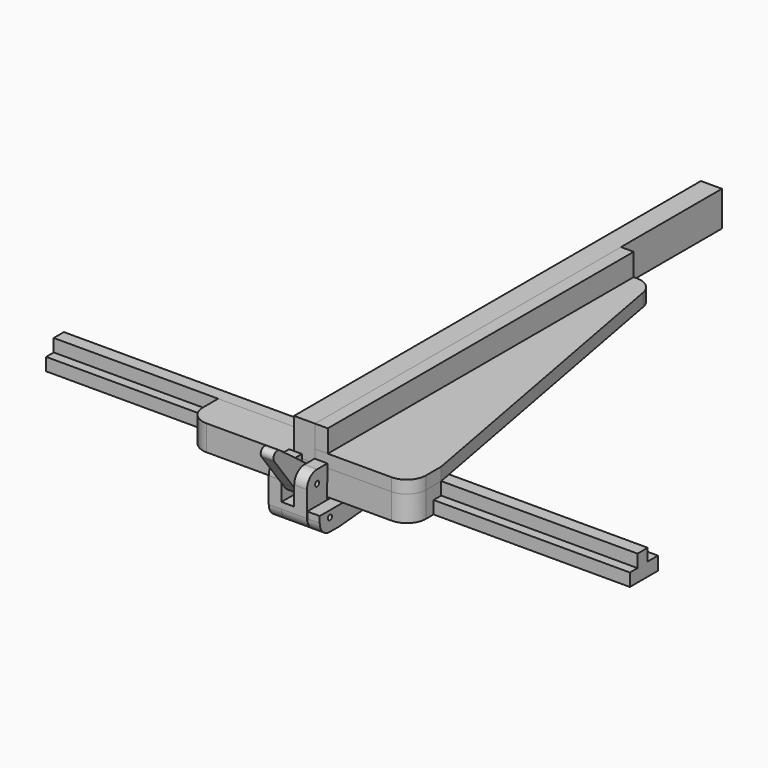
from build123d import *

# Parameters (mm, degrees)
F1_DEPTH      = 798
F2_W          = 150
F2_H          = 15
F3_DEPTH      = 20
F0_W          = 20
F0_H          = 35
F4_DEPTH      = 600
F2_W_2        = 200
F5_DEPTH      = 20
F6_DEPTH      = 40
F8_DEPTH      = 458
F8_DEPTH_BACK = 458
F7_R          = 5.125
F7_R_2        = 4
F9_DEPTH      = 20
F10_DEPTH     = 20
F11_START     = -40
F9_FACE_R     = 5.125
F9_FACE_R_2   = 4
F11_DEPTH     = 20
F12_DEPTH     = 20
F13_START     = 20.5
F13_DEPTH     = 19.5


with BuildPart() as f1:
    # F0 (on Front) → F1 (new body)
    with BuildSketch(Plane.XZ):
        Polygon((-33, 0), (0, 0), (0, 20), (0, 55), (-33, 55), align=None)
    extrude(amount=-F1_DEPTH)


with BuildPart() as f3:
    # F2 (on Top) → F3 (new body)
    with BuildSketch(Plane.XY):
        with BuildLine():
            Line((0, 600), (0, 60))
            Line((0, 60), (150, 60))
            Line((150, 60), (54.5439485545, 575.4626778055))
            ThreePointArc((54.5439485545, 575.4626778055), (44.2303739381, 593.0638281099), (25.045488405, 600))
            Line((25.045488405, 600), (0, 600))
        make_face()
        with BuildLine():
            Line((0, 45), (0, 0))
            Line((0, 0), (120, 0))
            ThreePointArc((120, 0), (141.2132034356, 8.7867965644), (150, 30))
            Line((150, 30), (150, 45))
            Line((150, 45), (0, 45))
        make_face()
        with Locations((75, 52.5)):
            Rectangle(F2_W, F2_H)
    extrude(amount=F3_DEPTH)


with BuildPart() as f4:
    # F0 (on Front) → F4 (new body, through all)
    with BuildSketch(Plane.XZ):
        with Locations((10, 37.5)):
            Rectangle(F0_W, F0_H)
    extrude(amount=-F4_DEPTH)


with BuildPart() as f5:
    # F2 (on Top) → F5 (new body)
    with BuildSketch(Plane.XY):
        with BuildLine():
            Line((0, 45), (0, 0))
            Line((0, 0), (120, 0))
            ThreePointArc((120, 0), (141.2132034356, 8.7867965644), (150, 30))
            Line((150, 30), (150, 45))
            Line((150, 45), (0, 45))
        make_face()
        with BuildLine():
            Line((-170, 0), (0, 0))
            Line((0, 0), (0, 45))
            Line((0, 45), (-200, 45))
            Line((-200, 45), (-200, 30))
            ThreePointArc((-200, 30), (-191.2132034356, 8.7867965644), (-170, 0))
        make_face()
        with Locations((-100, 52.5)):
            Rectangle(F2_W_2, F2_H)
        with Locations((75, 52.5)):
            Rectangle(F2_W, F2_H)
    extrude(amount=-F5_DEPTH)

    # F2 (on Top) → F6 (join)
    with BuildSketch(Plane.XY):
        with BuildLine():
            Line((-170, 0), (0, 0))
            Line((0, 0), (0, 45))
            Line((0, 45), (-200, 45))
            Line((-200, 45), (-200, 30))
            ThreePointArc((-200, 30), (-191.2132034356, 8.7867965644), (-170, 0))
        make_face()
        with BuildLine():
            Line((0, 45), (0, 0))
            Line((0, 0), (120, 0))
            ThreePointArc((120, 0), (141.2132034356, 8.7867965644), (150, 30))
            Line((150, 30), (150, 45))
            Line((150, 45), (0, 45))
        make_face()
    extrude(amount=-F6_DEPTH)


with BuildPart() as f8:
    # F7 (on Right) → F8 (new body, two sides)
    with BuildSketch(Plane.YZ) as f8_sk:
        Polygon((60, -20), (45, -20), (45, -40), (100, -40), (100, -19), (80, -19), (80, 0), (60, 0), align=None)
    extrude(amount=F8_DEPTH)
    extrude(f8_sk.sketch, amount=-F8_DEPTH_BACK)


with BuildPart() as f9:
    # F7 (on Right) → F9 (new body)
    with BuildSketch(Plane.YZ):
        with BuildLine():
            Line((100.7131075272, -43.0518470941), (-1.2868924728, -43.0518470941))
            Line((-1.2868924728, -43.0518470941), (-40.7868924728, -43.0518470941))
            Line((-40.7868924728, -43.0518470941), (-40.7868924728, -53.0518470941))
            ThreePointArc((-40.7868924728, -53.0518470941), (-34.9290280966, -67.1939827178), (-20.7868924728, -73.0518470941))
            Line((-20.7868924728, -73.0518470941), (-1.7868924728, -73.0518470941))
            Line((-1.7868924728, -73.0518470941), (100.7131075272, -64.0114742078))
            Line((100.7131075272, -64.0114742078), (100.7131075272, -43.0518470941))
        make_face()
        with Locations((-20.7868924728, -53.0518470941)):
            Circle(F7_R, mode=Mode.SUBTRACT)
        with BuildLine():
            ThreePointArc((-33.7822252527, -26.3080673665), (-15.8857687606, -33.5760469744), (-1.0682204113, -21.1846409416))
            Line((-1.0682204113, -21.1846409416), (-0.9491201788, -9.2746176901))
            ThreePointArc((-0.9491201788, -9.2746176901), (-3.5271920064, -4.1567086519), (-7.5306722004, -0.0565143142))
            Line((-7.5306722004, -0.0565143142), (-16.862163006, 6.9481529059))
            Line((-16.862163006, 6.9481529059), (-20.7868924728, 6.9481529059))
            ThreePointArc((-20.7868924728, 6.9481529059), (-34.9290280966, 1.0902885296), (-40.7868924728, -13.0518470941))
            Line((-40.7868924728, -13.0518470941), (-40.7868924728, -16.9765765609))
            Line((-40.7868924728, -16.9765765609), (-33.7822252527, -26.3080673665))
        make_face()
        with Locations((-20.7868924728, -13.0518470941)):
            Circle(F7_R_2, mode=Mode.SUBTRACT)
        with BuildLine():
            ThreePointArc((-7.5306722004, -0.0565143142), (-3.5271920064, -4.1567086519), (-0.9491201788, -9.2746176901))
            Line((-0.9491201788, -9.2746176901), (-0.7868924728, 6.9481529059))
            Line((-0.7868924728, 6.9481529059), (-16.862163006, 6.9481529059))
            Line((-16.862163006, 6.9481529059), (-7.5306722004, -0.0565143142))
        make_face()
        with BuildLine():
            Line((100.7131075272, -23.0518470941), (100.7131075272, -43.0518470941))
            Line((100.7131075272, -43.0518470941), (100.7131075272, -64.0114742078))
            Line((100.7131075272, -64.0114742078), (112.4702614954, -62.9745078083))
            ThreePointArc((112.4702614954, -62.9745078083), (125.4634139539, -56.5584551182), (130.7131075272, -43.0518470941))
            Line((130.7131075272, -43.0518470941), (130.7131075272, -33.0518470941))
            ThreePointArc((130.7131075272, -33.0518470941), (127.784175339, -25.9807792822), (120.7131075272, -23.0518470941))
            Line((120.7131075272, -23.0518470941), (100.7131075272, -23.0518470941))
        make_face()
        with BuildLine():
            Line((-40.7868924728, -43.0518470941), (-1.2868924728, -43.0518470941))
            Line((-1.2868924728, -43.0518470941), (-1.0682204113, -21.1846409416))
            ThreePointArc((-1.0682204113, -21.1846409416), (-15.8857687606, -33.5760469744), (-33.7822252527, -26.3080673665))
            Line((-33.7822252527, -26.3080673665), (-40.7868924728, -16.9765765609))
            Line((-40.7868924728, -16.9765765609), (-40.7868924728, -43.0518470941))
        make_face()
    extrude(amount=F9_DEPTH)

    # F7 (on Right) → F10 (join)
    with BuildSketch(Plane.YZ):
        with BuildLine():
            Line((100.7131075272, -43.0518470941), (-1.2868924728, -43.0518470941))
            Line((-1.2868924728, -43.0518470941), (-40.7868924728, -43.0518470941))
            Line((-40.7868924728, -43.0518470941), (-40.7868924728, -53.0518470941))
            ThreePointArc((-40.7868924728, -53.0518470941), (-34.9290280966, -67.1939827178), (-20.7868924728, -73.0518470941))
            Line((-20.7868924728, -73.0518470941), (-1.7868924728, -73.0518470941))
            Line((-1.7868924728, -73.0518470941), (100.7131075272, -64.0114742078))
            Line((100.7131075272, -64.0114742078), (100.7131075272, -43.0518470941))
        make_face()
        with Locations((-20.7868924728, -53.0518470941)):
            Circle(F7_R, mode=Mode.SUBTRACT)
    extrude(amount=-F10_DEPTH)

    # F9_face (on face) → F11 (join)
    with BuildSketch(Plane(origin=(20, 28.8911192498, -43.4988944495), x_dir=(0, 1, 0), z_dir=(1, 0, 0)).offset(F11_START)):
        with BuildLine():
            Line((-30.6780117226, -29.5529526446), (83.5791422456, -19.4756133588))
            ThreePointArc((83.5791422456, -19.4756133588), (96.5722947041, -13.0595606688), (101.8219882774, 0.4470473554))
            Line((101.8219882774, 0.4470473554), (101.8219882774, 10.4470473554))
            ThreePointArc((101.8219882774, 10.4470473554), (98.8930560892, 17.5181151673), (91.8219882774, 20.4470473554))
            Line((91.8219882774, 20.4470473554), (71.8219882774, 20.4470473554))
            Line((71.8219882774, 20.4470473554), (71.8219882774, 0.4470473554))
            Line((71.8219882774, 0.4470473554), (-30.1780117226, 0.4470473554))
            Line((-30.1780117226, 0.4470473554), (-29.6780117226, 50.4470473554))
            Line((-29.6780117226, 50.4470473554), (-49.6780117226, 50.4470473554))
            ThreePointArc((-49.6780117226, 50.4470473554), (-63.8201473463, 44.5891829791), (-69.6780117226, 30.4470473554))
            Line((-69.6780117226, 30.4470473554), (-69.6780117226, -9.5529526446))
            ThreePointArc((-69.6780117226, -9.5529526446), (-63.8201473463, -23.6950882683), (-49.6780117226, -29.5529526446))
            Line((-49.6780117226, -29.5529526446), (-30.6780117226, -29.5529526446))
        make_face()
        with Locations((-49.6780117226, -9.5529526446)):
            Circle(F9_FACE_R, mode=Mode.SUBTRACT)
        with Locations((-49.6780117226, 30.4470473554)):
            Circle(F9_FACE_R_2, mode=Mode.SUBTRACT)
    extrude(amount=-F11_DEPTH)


with BuildPart() as f12:
    # F7 (on Right) → F12 (new body)
    with BuildSketch(Plane.YZ):
        with BuildLine():
            ThreePointArc((-33.7822252527, -26.3080673665), (-15.8857687606, -33.5760469744), (-1.0682204113, -21.1846409416))
            Line((-1.0682204113, -21.1846409416), (-0.9491201788, -9.2746176901))
            ThreePointArc((-0.9491201788, -9.2746176901), (-3.5271920064, -4.1567086519), (-7.5306722004, -0.0565143142))
            Line((-7.5306722004, -0.0565143142), (-16.862163006, 6.9481529059))
            Line((-16.862163006, 6.9481529059), (-20.7868924728, 6.9481529059))
            ThreePointArc((-20.7868924728, 6.9481529059), (-34.9290280966, 1.0902885296), (-40.7868924728, -13.0518470941))
            Line((-40.7868924728, -13.0518470941), (-40.7868924728, -16.9765765609))
            Line((-40.7868924728, -16.9765765609), (-33.7822252527, -26.3080673665))
        make_face()
        with Locations((-20.7868924728, -13.0518470941)):
            Circle(F7_R_2, mode=Mode.SUBTRACT)
        with BuildLine():
            Line((-80.0382489084, 35.3133695813), (-40.7868924728, -16.9765765609))
            Line((-40.7868924728, -16.9765765609), (-40.7868924728, -13.0518470941))
            ThreePointArc((-40.7868924728, -13.0518470941), (-34.9290280966, 1.0902885296), (-20.7868924728, 6.9481529059))
            Line((-20.7868924728, 6.9481529059), (-16.862163006, 6.9481529059))
            Line((-16.862163006, 6.9481529059), (-69.1521091483, 46.1995093414))
            ThreePointArc((-69.1521091483, 46.1995093414), (-79.3179066679, 45.479167101), (-80.0382489084, 35.3133695813))
        make_face()
        with BuildLine():
            Line((-0.9491201788, -9.2746176901), (-1.0682204113, -21.1846409416))
            ThreePointArc((-1.0682204113, -21.1846409416), (-0.0378299025, -15.2393377198), (-0.9491201788, -9.2746176901))
        make_face()
    extrude(amount=-F12_DEPTH)


with BuildPart() as f13:
    # F7 (on Right) → F13 (new body)
    with BuildSketch(Plane.YZ.offset(F13_START)):
        with BuildLine():
            Line((100.7131075272, -43.0518470941), (-1.2868924728, -43.0518470941))
            Line((-1.2868924728, -43.0518470941), (-40.7868924728, -43.0518470941))
            Line((-40.7868924728, -43.0518470941), (-40.7868924728, -53.0518470941))
            ThreePointArc((-40.7868924728, -53.0518470941), (-34.9290280966, -67.1939827178), (-20.7868924728, -73.0518470941))
            Line((-20.7868924728, -73.0518470941), (-1.7868924728, -73.0518470941))
            Line((-1.7868924728, -73.0518470941), (100.7131075272, -64.0114742078))
            Line((100.7131075272, -64.0114742078), (100.7131075272, -43.0518470941))
        make_face()
        with Locations((-20.7868924728, -53.0518470941)):
            Circle(F7_R, mode=Mode.SUBTRACT)
        with Locations((-20.7868924728, -53.0518470941)):
            Circle(F7_R)
        with Locations((-20.7868924728, -53.0518470941)):
            Circle(F7_R_2, mode=Mode.SUBTRACT)
    extrude(amount=F13_DEPTH)


solid = Compound([f1.part, f3.part, f4.part, f5.part, f8.part, f9.part, f12.part, f13.part])
